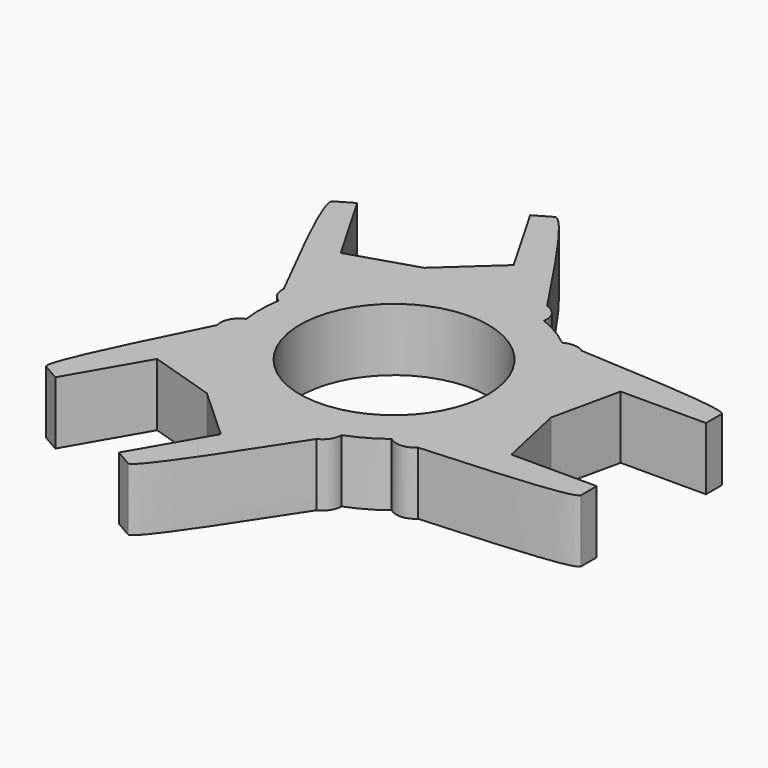
from build123d import *

# Parameters (mm, degrees)
F0_R     = 9.525
F1_DEPTH = 6.35
F3_COUNT = 3
F4_R     = 9.525
F5_DEPTH = 6.35
F7_DEPTH = 6.35


with BuildPart() as f1:
    # F0 (on Top) → F1 (new body)
    with BuildSketch(Plane.XY):
        with BuildLine():
            Line((9.525, 0), (12.7, 0))
            ThreePointArc((12.7, 0), (12.1234798492, 3.7830194747), (10.4462619928, 7.2225764363))
            ThreePointArc((10.4462619928, 7.2225764363), (10.00070112, 7.0453500483), (9.525, 6.985))
            Line((9.525, 6.985), (9.525, 0))
        make_face()
        with BuildLine():
            ThreePointArc((9.525, -8.4002604126), (9.9057858228, -7.9476667791), (10.2650859452, -7.4778346155))
            ThreePointArc((10.2650859452, -7.4778346155), (9.9025309799, -7.3659812593), (9.525, -7.3281971973))
            Line((9.525, -7.3281971973), (9.525, -8.4002604126))
        make_face()
        with BuildLine():
            ThreePointArc((11.3988304843, -8.89), (11.0104940402, -8.040581393), (10.2650859452, -7.4778346155))
            ThreePointArc((10.2650859452, -7.4778346155), (9.9057858228, -7.9476667791), (9.525, -8.4002604126))
            Line((9.525, -8.4002604126), (9.525, -8.89))
            Line((9.525, -8.89), (11.3988304843, -8.89))
        make_face()
        with BuildLine():
            ThreePointArc((7.7935067776, -10.0275247248), (8.6973942383, -9.2544764013), (9.525, -8.4002604126))
            Line((9.525, -8.4002604126), (9.525, -7.3281971973))
            ThreePointArc((9.525, -7.3281971973), (7.921532049, -8.2046469895), (7.7935067776, -10.0275247248))
        make_face()
        with BuildLine():
            Line((9.525, 6.985), (9.525, 8.4002604126))
            ThreePointArc((9.525, 8.4002604126), (8.7581956911, 9.196956466), (7.9249969146, 9.9239318772))
            ThreePointArc((7.9249969146, 9.9239318772), (7.8518793788, 7.9791254823), (9.525, 6.985))
        make_face()
        with BuildLine():
            ThreePointArc((10.4462619928, 7.2225764363), (12.1234798492, 3.7830194747), (12.7, 0))
            Line((12.7, 0), (15.875, 0))
            Line((15.875, 0), (17.399, 6.9088))
            Line((17.399, 6.9088), (26.035, 6.9088))
            Line((26.035, 6.9088), (26.035, 8.89))
            Line((26.035, 8.89), (11.43, 8.89))
            ThreePointArc((11.43, 8.89), (11.1657359776, 7.922006998), (10.4462619928, 7.2225764363))
        make_face()
        with BuildLine():
            ThreePointArc((9.525, 6.985), (10.00070112, 7.0453500483), (10.4462619928, 7.2225764363))
            ThreePointArc((10.4462619928, 7.2225764363), (10.0029776208, 7.8249880969), (9.525, 8.4002604126))
            Line((9.525, 8.4002604126), (9.525, 6.985))
        make_face()
        with BuildLine():
            ThreePointArc((9.525, 8.4002604126), (10.0029776208, 7.8249880969), (10.4462619928, 7.2225764363))
            ThreePointArc((10.4462619928, 7.2225764363), (11.1657359776, 7.922006998), (11.43, 8.89))
            Line((11.43, 8.89), (9.525, 8.89))
            Line((9.525, 8.89), (9.525, 8.4002604126))
        make_face()
        with BuildLine():
            Line((9.525, -8.89), (9.525, -8.4002604126))
            ThreePointArc((9.525, -8.4002604126), (8.6973942383, -9.2544764013), (7.7935067776, -10.0275247248))
            ThreePointArc((7.7935067776, -10.0275247248), (9.9315282348, -11.0943150857), (11.43, -9.2331971973))
            ThreePointArc((11.43, -9.2331971973), (11.4221916182, -9.0608923403), (11.3988304843, -8.89))
            Line((11.3988304843, -8.89), (9.525, -8.89))
        make_face()
        with BuildLine():
            ThreePointArc((7.9249969146, 9.9239318772), (8.7581956911, 9.196956466), (9.525, 8.4002604126))
            Line((9.525, 8.4002604126), (9.525, 8.89))
            Line((9.525, 8.89), (11.43, 8.89))
            ThreePointArc((11.43, 8.89), (10.0639893887, 10.7171604852), (7.9249969146, 9.9239318772))
        make_face()
        with BuildLine():
            Line((15.875, 0), (12.7, 0))
            ThreePointArc((12.7, 0), (12.075938711, -3.9321373638), (10.2650859452, -7.4778346155))
            ThreePointArc((10.2650859452, -7.4778346155), (11.0104940402, -8.040581393), (11.3988304843, -8.89))
            Line((11.3988304843, -8.89), (26.035, -8.89))
            Line((26.035, -8.89), (26.035, -6.9088))
            Line((26.035, -6.9088), (17.399, -6.9088))
            Line((17.399, -6.9088), (15.875, 0))
        make_face()
        with BuildLine():
            ThreePointArc((10.2650859452, -7.4778346155), (12.075938711, -3.9321373638), (12.7, 0))
            Line((12.7, 0), (9.525, 0))
            Line((9.525, 0), (9.525, -7.3281971973))
            ThreePointArc((9.525, -7.3281971973), (9.9025309799, -7.3659812593), (10.2650859452, -7.4778346155))
        make_face()
        with BuildLine():
            Line((9.525, -7.3281971973), (9.525, 0))
            Line((9.525, 0), (9.525, 6.985))
            ThreePointArc((9.525, 6.985), (7.8518793788, 7.9791254823), (7.9249969146, 9.9239318772))
            ThreePointArc((7.9249969146, 9.9239318772), (-12.6997241984, 0.0836975719), (7.7935067776, -10.0275247248))
            ThreePointArc((7.7935067776, -10.0275247248), (7.921532049, -8.2046469895), (9.525, -7.3281971973))
        make_face()
        Circle(F0_R, mode=Mode.SUBTRACT)
    extrude(amount=F1_DEPTH)


with BuildPart() as f3_1:
    # F3: instance of F1
    add(f1.part.rotate(Axis((0, 0, 3.175), (0, 0, 1)), 1 * 360 / F3_COUNT))


with BuildPart() as f3_2:
    # F3: instance of F1
    add(f1.part.rotate(Axis((0, 0, 3.175), (0, 0, 1)), 2 * 360 / F3_COUNT))


with BuildPart() as f1_1:
    add(f1.part)

    add(f3_1.part)  # F5 merges F3_1

    add(f3_2.part)  # F5 merges F3_2
    # F4 (on face) → F5 (join)
    with BuildSketch(Plane.XY.offset(6.35)):
        with BuildLine():
            ThreePointArc((4.8414628101, -12.6972894296), (11.1904325012, -7.7094190078), (13.589, 0))
            ThreePointArc((13.589, 0), (-0.9329227135, 13.5569383052), (-13.4609045126, -1.8614431777))
            ThreePointArc((-13.4609045126, -1.8614431777), (-13.0283174584, -1.7464719499), (-12.5808445376, -1.7356124916))
            ThreePointArc((-12.5808445376, -1.7356124916), (6.4223463228, 10.9564349909), (4.6318786538, -11.8252145916))
            ThreePointArc((4.6318786538, -11.8252145916), (4.7887256176, -12.2487417548), (4.8414628101, -12.6972894296))
        make_face()
        with BuildLine():
            ThreePointArc((-12.5808445376, -1.7356124916), (-13.0283174584, -1.7464719499), (-13.4609045126, -1.8614431777))
            ThreePointArc((-13.4609045126, -1.8614431777), (-6.9229751419, -11.6933030486), (4.8414628101, -12.6972894296))
            ThreePointArc((4.8414628101, -12.6972894296), (4.7887256176, -12.2487417548), (4.6318786538, -11.8252145916))
            ThreePointArc((4.6318786538, -11.8252145916), (6.4223463228, 10.9564349909), (-12.5808445376, -1.7356124916))
        make_face()
        Circle(F4_R, mode=Mode.SUBTRACT)
    extrude(amount=-F5_DEPTH)

    # F6 (on face) → F7 (join)
    with BuildSketch(Plane.XY.offset(6.35)):
        with BuildLine():
            add(Edge.make_bspline(
                [(10.6367632499, 10.4369348649), (18.6027915748, 10.0299773304), (25.9883071623, 9.6007507753), (26.035, 8.89)],
                knots=[0.0462368838, 0.0462368838, 0.0462368838, 0.0462368838, 0.584525149, 0.584525149, 0.584525149, 0.584525149], degree=3))
            ThreePointArc((10.6367632499, 10.4369348649), (11.2201303771, 9.7592283961), (11.43, 8.89))
            Line((11.43, 8.89), (26.035, 8.89))
        make_face()
        with BuildLine():
            ThreePointArc((1.9995505975, 14.3166767728), (2.8133537712, 14.7235401011), (3.7230379132, 14.7065655527))
            add(Edge.make_bspline(
                [(3.7230379132, 14.7065655527), (-0.6351401044, 21.3148502374), (-4.6685883244, 27.3160665919), (-5.3185341604, 26.9919713875)],
                knots=[0.0562643988, 0.0562643988, 0.0562643988, 0.0562643988, 0.5862434824, 0.5862434824, 0.5862434824, 0.5862434824], degree=3))
            Line((-5.3185341604, 26.9919713875), (1.9995505975, 14.3166767728))
        make_face()
        with BuildLine():
            add(Edge.make_bspline(
                [(10.8747404145, -10.5775281884), (18.7767718356, -10.1073776533), (25.9907017622, -9.6149172072), (26.035, -8.89)],
                knots=[0.0562643988, 0.0562643988, 0.0562643988, 0.0562643988, 0.5862434824, 0.5862434824, 0.5862434824, 0.5862434824], degree=3))
            Line((26.035, -8.89), (11.3988304843, -8.89))
            ThreePointArc((11.3988304843, -8.89), (11.3442828756, -9.7982058862), (10.8747404145, -10.5775281884))
        make_face()
        with BuildLine():
            Line((-13.4139658396, 5.4536703653), (-20.7164658396, 18.1019713875))
            add(Edge.make_bspline(
                [(-14.3570323556, 3.993239756), (-17.987610955, 11.0955014199), (-21.3086476479, 17.7061588163), (-20.7164658396, 18.1019713875)],
                knots=[0.0462368838, 0.0462368838, 0.0462368838, 0.0462368838, 0.584525149, 0.584525149, 0.584525149, 0.584525149], degree=3))
            ThreePointArc((-14.3570323556, 3.993239756), (-14.0618049009, 4.8373037423), (-13.4139658396, 5.4536703653))
        make_face()
        with BuildLine():
            add(Edge.make_bspline(
                [(3.7202691057, -14.4301746209), (-0.6151806199, -21.1254787503), (-4.6796595144, -27.3069095915), (-5.3185341604, -26.9919713875)],
                knots=[0.0462368838, 0.0462368838, 0.0462368838, 0.0462368838, 0.584525149, 0.584525149, 0.584525149, 0.584525149], degree=3))
            ThreePointArc((3.7202691057, -14.4301746209), (2.8416745238, -14.5965321384), (1.9839658396, -14.3436703653))
            Line((1.9839658396, -14.3436703653), (-5.3185341604, -26.9919713875))
        make_face()
        with BuildLine():
            ThreePointArc((-13.3983810818, -5.4266767728), (-14.1576366468, -4.9253342149), (-14.5977783276, -4.1290373643))
            add(Edge.make_bspline(
                [(-14.5977783276, -4.1290373643), (-18.1416317312, -11.207472584), (-21.3221134379, -17.7011493846), (-20.7164658396, -18.1019713875)],
                knots=[0.0562643988, 0.0562643988, 0.0562643988, 0.0562643988, 0.5862434824, 0.5862434824, 0.5862434824, 0.5862434824], degree=3))
            Line((-20.7164658396, -18.1019713875), (-13.3983810818, -5.4266767728))
        make_face()
    extrude(amount=-F7_DEPTH)


solid = f1_1.part
